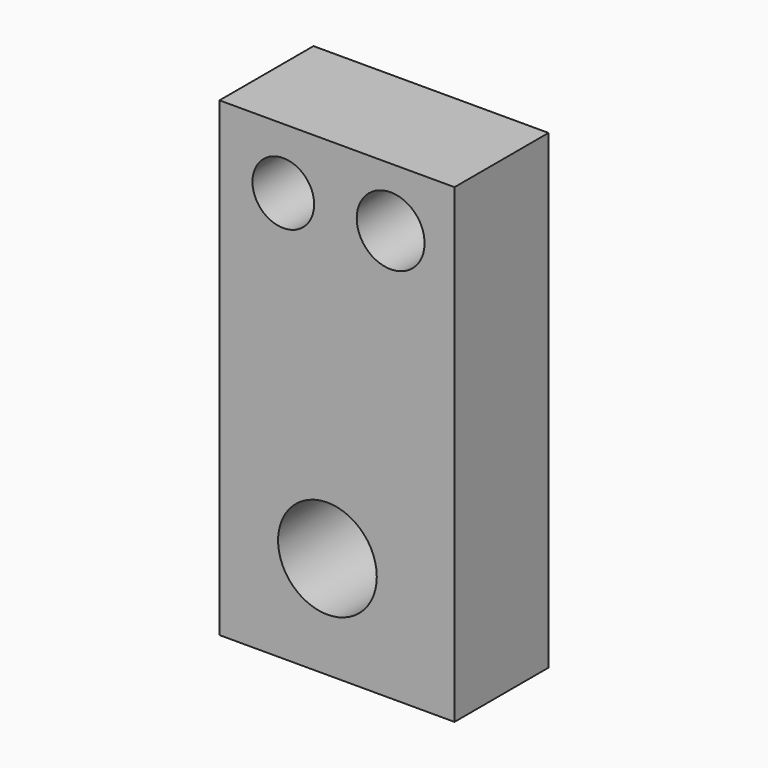
from build123d import *

# Parameters (mm, degrees)
F0_W     = 25.4605272785
F0_H     = 12.7302636392
F1_DEPTH = 51
F2_R     = 3.6756964622
F3_DEPTH = 25
F4_R     = 3.3400093655
F5_DEPTH = 25
F6_R     = 5.3474190326
F7_DEPTH = 25


# Not quite as in the source:
# - a feature names something its author has since deleted; it is built from what else it names


with BuildPart() as f1:
    # F0 (on Top) → F1 (new body)
    with BuildSketch(Plane.XY):
        with Locations((1.0361843742, 1.1842104141)):
            Rectangle(F0_W, F0_H)
    extrude(amount=F1_DEPTH)

    # F2 (on face) → F3 (cut)
    with BuildSketch(Plane(origin=(0, 7.5493422337, 0), x_dir=(-1, 0, 0), z_dir=(0, 1, 0))):
        with Locations((-6.8494305015, 44.5928275585)):
            Circle(F2_R)
    extrude(amount=-F3_DEPTH, mode=Mode.SUBTRACT)

    # F4 (on face) → F5 (cut)
    with BuildSketch(Plane(origin=(0, 7.5493422337, 0), x_dir=(-1, 0, 0), z_dir=(0, 1, 0))):
        with Locations((4.7804336064, 44.4043427706)):
            Circle(F4_R)
    extrude(amount=-F5_DEPTH, mode=Mode.SUBTRACT)

    # F6 (on face) → F7 (cut)
    with BuildSketch(Plane.XZ.offset(5.1809214056)):
        with Locations((0, 11.1019741744)):
            Circle(F6_R)
    extrude(amount=-F7_DEPTH, mode=Mode.SUBTRACT)


solid = f1.part
